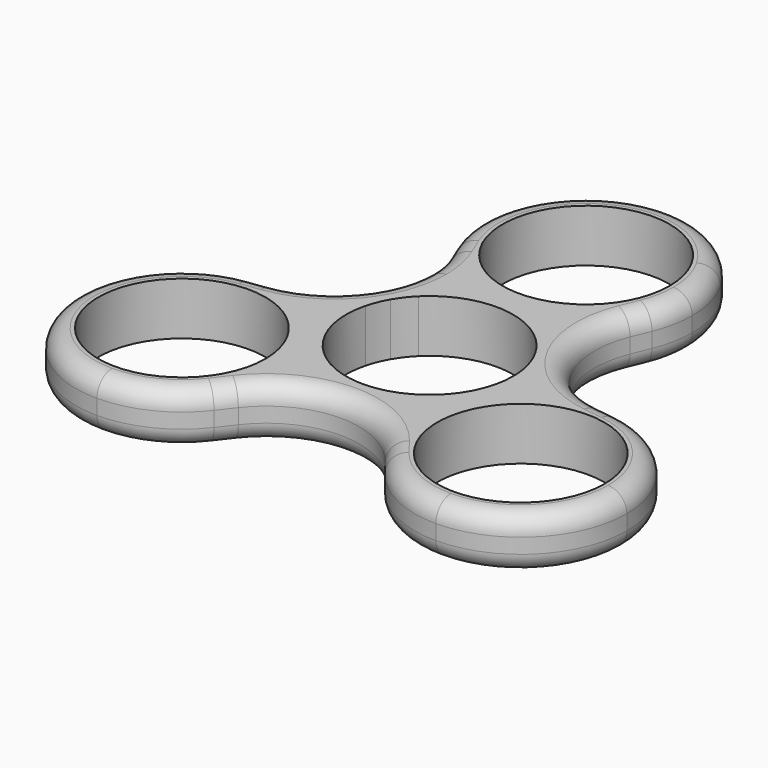
from build123d import *

# Parameters (mm, degrees)
F0_R     = 11.1
F1_DEPTH = 7
F2_R     = 2.5


with BuildPart() as f1:
    # F0 (on Top) → F1 (new body)
    with BuildSketch(Plane.XY):
        with BuildLine():
            ThreePointArc((10.7379469842, 2.8118489582), (11.0091146675, 1.4175310358), (11.1, 0))
            ThreePointArc((11.1, 0), (8.8254074573, -6.7321752214), (2.9338408627, -10.705259352))
            Line((2.9338408627, -10.705259352), (9.7685135139, -19.5601115638))
            Line((9.7685135139, -19.5601115638), (11.3548395287, -21.6153208089))
            ThreePointArc((11.3548395287, -21.6153208089), (10.305702305, -5.95), (24.3968366958, 0.9740809167))
            Line((24.3968366958, 0.9740809167), (21.8238104233, 1.3202749012))
            Line((21.8238104233, 1.3202749012), (10.7379469842, 2.8118489582))
        make_face()
        with BuildLine():
            ThreePointArc((9.612881982, 5.55), (10.2671041528, 4.2185983827), (10.7379469842, 2.8118489582))
            Line((10.7379469842, 2.8118489582), (21.8238104233, 1.3202749012))
            ThreePointArc((21.8238104233, 1.3202749012), (12.7825990769, 7.3800369283), (12.0552967571, 18.2398366397))
            Line((12.0552967571, 18.2398366397), (7.8041061216, 7.8934103937))
            ThreePointArc((7.8041061216, 7.8934103937), (8.7869654442, 6.7822738283), (9.612881982, 5.55))
        make_face()
        with BuildLine():
            Line((9.7685135139, -19.5601115638), (2.9338408627, -10.705259352))
            ThreePointArc((2.9338408627, -10.705259352), (1.4801387086, -11.000872211), (0, -11.1))
            ThreePointArc((0, -11.1), (-1.4801387086, -11.000872211), (-2.9338408627, -10.705259352))
            Line((-2.9338408627, -10.705259352), (-9.7685137049, -19.5601118111))
            ThreePointArc((-9.7685137049, -19.5601118111), (-1.562e-07, -14.7600739912), (9.7685135139, -19.5601115638))
        make_face()
        with BuildLine():
            ThreePointArc((-7.8041061216, 7.8934103937), (0, 11.1), (7.8041061216, 7.8934103937))
            Line((7.8041061216, 7.8934103937), (12.0552967571, 18.2398366397))
            Line((12.0552967571, 18.2398366397), (13.0419971671, 20.6412398922))
            ThreePointArc((13.0419971671, 20.6412398922), (0, 11.9), (-13.0419971671, 20.6412398922))
            Line((-13.0419971671, 20.6412398922), (-12.0552968552, 18.2398368784))
            Line((-12.0552968552, 18.2398368784), (-7.8041061216, 7.8934103937))
        make_face()
        with BuildLine():
            ThreePointArc((34.7276186918, -5.95), (30.3668669441, -1.2874315899), (24.3968366958, 0.9740809167))
            ThreePointArc((24.3968366958, 0.9740809167), (10.305702305, -5.95), (11.3548395287, -21.6153208089))
            ThreePointArc((11.3548395287, -21.6153208089), (16.2983819346, -25.6547624119), (22.5166604984, -27.1))
            ThreePointArc((22.5166604984, -27.1), (32.4868661131, -22.9702056147), (36.6166604984, -13))
            ThreePointArc((36.6166604984, -13), (36.1362146491, -9.3506514641), (34.7276186918, -5.95))
        make_face()
        with Locations((22.5166604984, -13)):
            Circle(F0_R, mode=Mode.SUBTRACT)
        with BuildLine():
            Line((-9.7685137049, -19.5601118111), (-2.9338408627, -10.705259352))
            ThreePointArc((-2.9338408627, -10.705259352), (-9.612881982, -5.55), (-10.7379469842, 2.8118489582))
            Line((-10.7379469842, 2.8118489582), (-21.8238108007, 1.3202748505))
            Line((-21.8238108007, 1.3202748505), (-24.3968366958, 0.9740809167))
            ThreePointArc((-24.3968366958, 0.9740809167), (-13.2349711151, -2.3858470808), (-8.4166604984, -13))
            ThreePointArc((-8.4166604984, -13), (-9.1714052428, -17.551281376), (-11.3548395287, -21.6153208089))
            Line((-11.3548395287, -21.6153208089), (-9.7685137049, -19.5601118111))
        make_face()
        with BuildLine():
            ThreePointArc((-9.612881982, 5.55), (-8.7869654442, 6.7822738283), (-7.8041061216, 7.8934103937))
            Line((-7.8041061216, 7.8934103937), (-12.0552968552, 18.2398368784))
            ThreePointArc((-12.0552968552, 18.2398368784), (-11.3630589396, 15.9401843286), (-11.1293624337, 13.55))
            ThreePointArc((-11.1293624337, 13.55), (-14.1800784048, 5.4269247956), (-21.8238108007, 1.3202748505))
            Line((-21.8238108007, 1.3202748505), (-10.7379469842, 2.8118489582))
            ThreePointArc((-10.7379469842, 2.8118489582), (-10.2671041528, 4.2185983827), (-9.612881982, 5.55))
        make_face()
        with BuildLine():
            ThreePointArc((-13.0419971671, 20.6412398922), (0, 11.9), (13.0419971671, 20.6412398922))
            ThreePointArc((13.0419971671, 20.6412398922), (13.8329707593, 23.2688976636), (14.1, 26))
            ThreePointArc((14.1, 26), (13.6195541507, 29.6493485359), (12.2109581934, 33.05))
            ThreePointArc((12.2109581934, 33.05), (0, 40.1), (-12.2109581934, 33.05))
            ThreePointArc((-12.2109581934, 33.05), (-14.0684850095, 26.9421940019), (-13.0419971671, 20.6412398922))
        make_face()
        with Locations((0, 26)):
            Circle(F0_R, mode=Mode.SUBTRACT)
        with BuildLine():
            ThreePointArc((-22.5166604984, -27.1), (-16.2983819346, -25.6547624119), (-11.3548395287, -21.6153208089))
            ThreePointArc((-11.3548395287, -21.6153208089), (-9.1714052428, -17.551281376), (-8.4166604984, -13))
            ThreePointArc((-8.4166604984, -13), (-13.2349711151, -2.3858470808), (-24.3968366958, 0.9740809167))
            ThreePointArc((-24.3968366958, 0.9740809167), (-30.3668669441, -1.2874315899), (-34.7276186918, -5.95))
            ThreePointArc((-34.7276186918, -5.95), (-34.7276186918, -20.05), (-22.5166604984, -27.1))
        make_face()
        with Locations((-22.5166604984, -13)):
            Circle(F0_R, mode=Mode.SUBTRACT)
    extrude(amount=F1_DEPTH)

    # F2
    f2_edges = [f1.edges().sort_by_distance(p)[0] for p in [
        (-34.727619, -20.05, 7),
        (-34.727619, -20.05, 0),
        (10.561677, -20.587716, 0),
        (10.561677, -20.587716, 7),
        (34.727619, -20.05, 0),
        (34.727619, -20.05, 7),
        (23.110324, 1.147178, 0),
        (23.110324, 1.147178, 7),
        (12.782599, 7.380037, 0),
        (12.782599, 7.380037, 7),
        (12.548647, 19.440538, 0),
        (12.548647, 19.440538, 7),
        (0, 40.1, 0),
        (0, 40.1, 7),
        (-12.548647, 19.440538, 0),
        (-12.548647, 19.440538, 7),
        (-12.782599, 7.380037, 0),
        (-12.782599, 7.380037, 7),
        (-23.110324, 1.147178, 0),
        (-23.110324, 1.147178, 7),
        (-10.561677, -20.587716, 0),
        (-10.561677, -20.587716, 7),
        (0, -14.760074, 0),
        (0, -14.760074, 7),
    ]]
    fillet(f2_edges, radius=F2_R)


solid = f1.part
